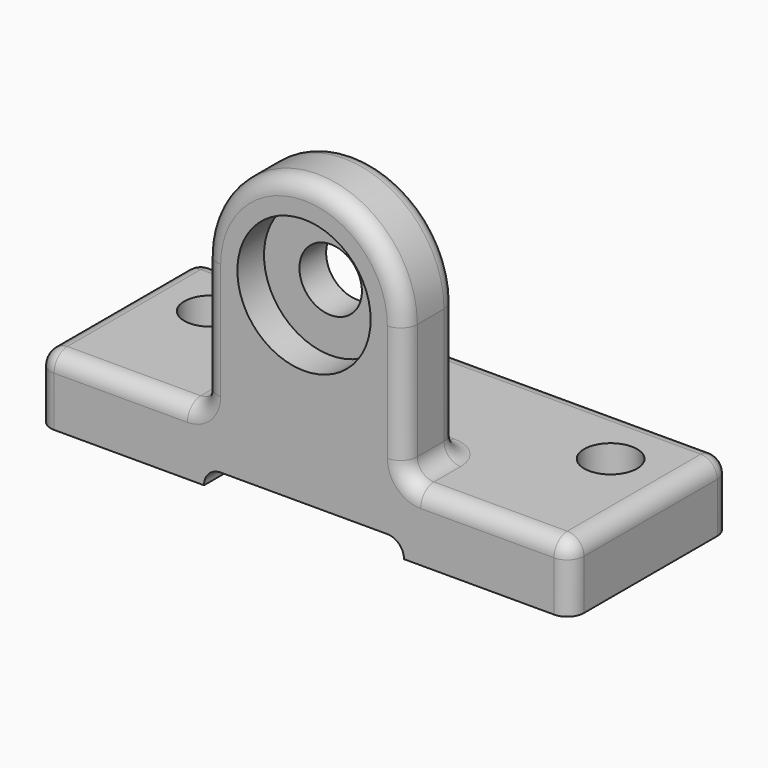
from build123d import *

# Parameters (mm, degrees)
F0_W           = 101.6
F0_H           = 38.1
F1_DEPTH       = 12.7
F3_DEPTH       = 12.7
F5_D           = 11.90625
F5_CBORE_D     = 25.4
F5_CBORE_DEPTH = 6.35
F6_W           = 38.1
F6_H           = 3.175
F7_DEPTH       = 38.101
F9_D           = 10.0838
F10_R          = 3.17499
F11_R          = 3.17499


# Not quite as in the source:
# - a fillet or chamfer is up to 0.001 mm smaller than in the source, because OpenCascade refuses the exact size
# - a length typed as a fraction of an inch, garbled in the dataset ("3 / 203.2 mm" for 3/8 in), is restored


with BuildPart() as f1:
    # F0 (on Top) → F1 (new body)
    with BuildSketch(Plane.XY):
        with Locations((50.8, 19.05)):
            Rectangle(F0_W, F0_H)
    extrude(amount=F1_DEPTH)

    # F2 (on Front) → F3 (join)
    with BuildSketch(Plane.XZ):
        with BuildLine():
            Line((31.75, 38.1), (31.75, 0))
            Line((31.75, 0), (69.85, 0))
            Line((69.85, 0), (69.85, 38.1))
            ThreePointArc((69.85, 38.1), (50.8, 57.15), (31.75, 38.1))
        make_face()
    extrude(amount=-F3_DEPTH)

    # F5 (through all)
    with Locations(Plane.XZ):
        with Locations((50.8, 38.1)):
            CounterBoreHole(F5_D / 2, F5_CBORE_D / 2, F5_CBORE_DEPTH)

    # F6 (on face) → F7 (cut, through all)
    with BuildSketch(Plane.XZ):
        with Locations((50.8, 1.5875)):
            Rectangle(F6_W, F6_H)
    extrude(amount=-F7_DEPTH, mode=Mode.SUBTRACT)

    # F9 (through all)
    with Locations(Plane.XY.offset(12.7)):
        with Locations((12.7, 25.4), (88.9, 25.4)):
            Hole(F9_D / 2)

    # F10 (radius 3.175 in the source; OpenCascade refuses exactly that, so slightly less here)
    f10_edges = [f1.edges().sort_by_distance(p)[0] for p in [
        (0, 0, 6.35),
        (0, 38.1, 6.35),
        (101.6, 0, 6.35),
        (101.6, 38.1, 6.35),
        (31.75, 19.05, 3.175),
        (69.85, 19.05, 3.175),
    ]]
    fillet(f10_edges, radius=F10_R)

    # F11 (radius 3.175 in the source; OpenCascade refuses exactly that, so slightly less here)
    f11_edges = [f1.edges().sort_by_distance(p)[0] for p in [
        (50.8, 38.1, 12.7),
        (101.6, 19.05, 12.7),
        (100.670067, 37.170067, 12.7),
        (100.670067, 0.929933, 12.7),
        (84.137505, 0, 12.7),
        (0.929933, 37.170067, 12.7),
        (0, 19.05, 12.7),
        (0.929933, 0.929933, 12.7),
        (17.462495, 0, 12.7),
        (31.75, 0, 25.4),
        (50.8, 0, 57.15),
        (69.85, 0, 25.4),
        (69.85, 6.35, 12.7),
        (31.75, 6.35, 12.7),
        (50.8, 12.7, 12.7),
        (31.75, 12.7, 25.4),
        (50.8, 12.7, 57.15),
        (69.85, 12.7, 25.4),
    ]]
    fillet(f11_edges, radius=F11_R)


solid = f1.part
